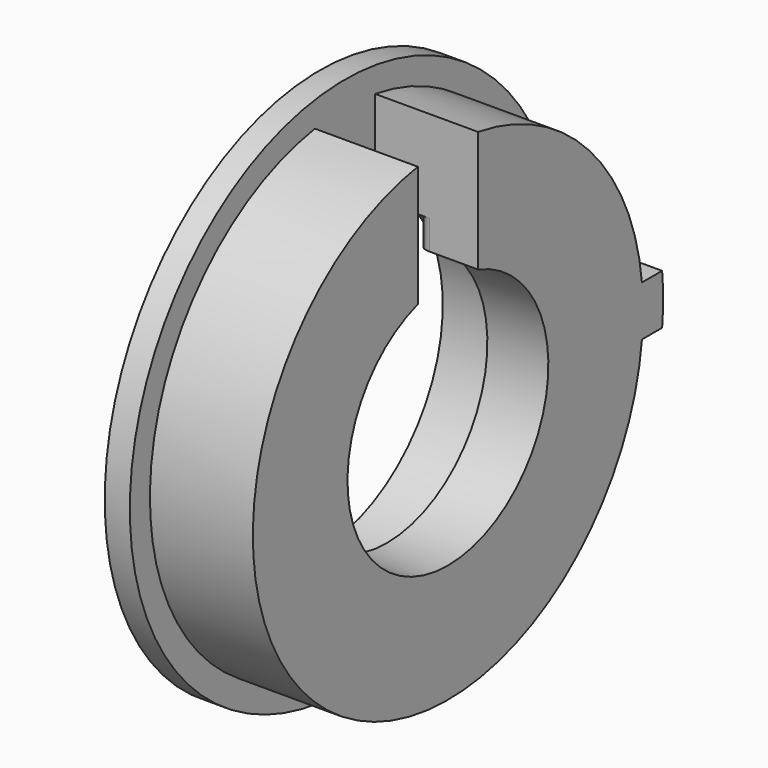
from build123d import *

# Parameters (mm, degrees)
F0_R      = 21.4215
F1_DEPTH  = 10.2
F3_DEPTH  = 8.2
F4_R      = 12.24
F5_DEPTH  = 5.344
F6_W      = 8.2
F6_H      = 6
F7_DEPTH  = 25
F8_R      = 1
F9_R      = 10
F10_DEPTH = 6


with BuildPart() as f1:
    # F0 (on Right) → F1 (new body)
    with BuildSketch(Plane.YZ):
        Circle(F0_R)
    extrude(amount=-F1_DEPTH)

    # F2 (on face) → F3 (cut)
    with BuildSketch(Plane.YZ):
        with BuildLine():
            ThreePointArc((19.3182468731, -2), (-19.4215, 0), (19.3182468731, 2))
            Line((19.3182468731, 2), (21.3279315043, 2))
            ThreePointArc((21.3279315043, 2), (-21.4215, 0), (21.3279315043, -2))
            Line((21.3279315043, -2), (19.3182468731, -2))
        make_face()
    extrude(amount=-F3_DEPTH, mode=Mode.SUBTRACT)

    # F4 (on face) → F5 (cut)
    with BuildSketch(Plane(origin=(-10.2, 0, 0), x_dir=(0, -1, 0), z_dir=(-1, 0, 0))):
        Circle(F4_R)
    extrude(amount=-F5_DEPTH, mode=Mode.SUBTRACT)

    # F6 (on Top) → F7 (cut)
    with BuildSketch(Plane.XY):
        with Locations((-4.1, 0)):
            Rectangle(F6_W, F6_H)
    extrude(amount=F7_DEPTH, mode=Mode.SUBTRACT)

    # F8
    f8_edges = [f1.edges().sort_by_distance(p)[0] for p in [
        (-4.856, 3, 5.93333),
        (-4.856, -3, 5.93333),
        (-8.2, 0, 12.24),
    ]]
    fillet(f8_edges, radius=F8_R)

    # F9 (on face) → F10 (cut)
    with BuildSketch(Plane.YZ):
        Circle(F9_R)
    extrude(amount=-F10_DEPTH, mode=Mode.SUBTRACT)


solid = f1.part
